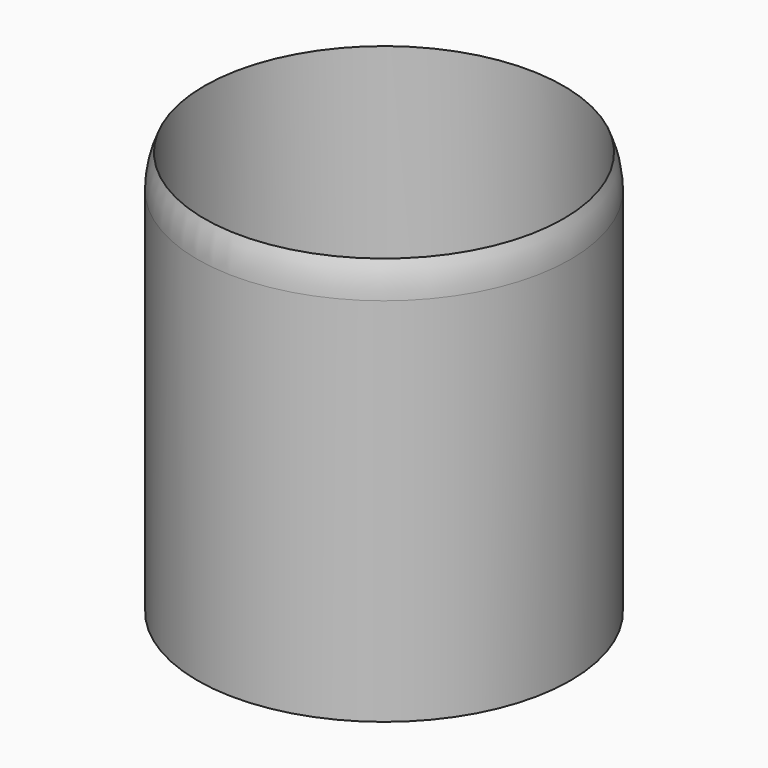
from build123d import *

# Parameters (mm, degrees)
F0_R     = 68.5822054127
F1_DEPTH = 148.59
F2_T     = -2.54


# Not quite as in the source:
# - a fillet or chamfer that OpenCascade refuses, or shapes differently, is made with other operations: its cross-section is extruded or revolved along the edge and cut away or added


with BuildPart() as f1:
    # F0 (on Top) → F1 (new body)
    with BuildSketch(Plane.XY):
        Circle(F0_R)
    extrude(amount=-F1_DEPTH)

    # F2
    f2_openings = [f1.faces().sort_by_distance(p)[0] for p in [
        (0, 0, 0),
    ]]
    offset(amount=F2_T, openings=f2_openings)

    # F3: fillet of radius 31.273722487 on 1 edges, made by hand

    # F3_s1 → F3_t2 (revolve, cut)
    with BuildSketch(Plane.XZ):
        with BuildLine():
            ThreePointArc((68.5822054127, -12.34580537), (67.9406243892, -6.0436130881), (66.0422054127, 0))
            Line((66.0422054127, 0), (66.6168798625, 0.2469161074))
            ThreePointArc((66.6168798625, 0.2469161074), (67.3122054127, 0.6254744497), (68.5822054127, 0.6254744497))
            Line((68.5822054127, 0.6254744497), (69.2076798625, 0))
            Line((69.2076798625, 0), (69.2076798625, -12.34580537))
            Line((69.2076798625, -12.34580537), (68.5822054127, -12.34580537))
        make_face()
    revolve(axis=Axis((0, 0, 0), (0, 0, 1)), mode=Mode.SUBTRACT)


solid = f1.part
